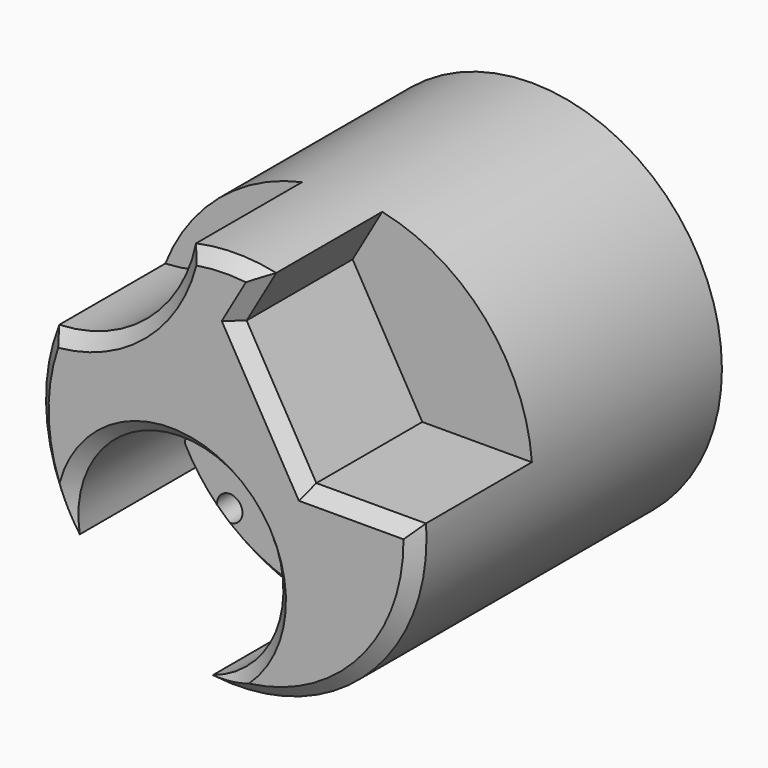
from build123d import *

# Parameters (mm, degrees)
F0_R        = 37.9287365184
F1_DEPTH    = 76.2
F3_R        = 20.4430640503
F4_DEPTH    = 43.688
F5_SIZE     = 2.54
F7_D        = 5.08
F8_T4_ANGLE = 68.0337710329
F8_S5_R     = 20.4430640503
F8_T6_DEPTH = 23


# Not quite as in the source:
# - a fillet or chamfer that OpenCascade refuses, or shapes differently, is made with other operations: its cross-section is extruded or revolved along the edge and cut away or added


with BuildPart() as f1:
    # F0 (on Front) → F1 (new body)
    with BuildSketch(Plane.XZ):
        Circle(F0_R)
    extrude(amount=F1_DEPTH)

    # F3 (on offset) → F4 (cut)
    with BuildSketch(Plane.XZ.offset(47.244)):
        with BuildLine():
            Line((-7.417100016, 52.0775169134), (-39.2948538065, 52.0775169134))
            Line((-39.2948538065, 52.0775169134), (-39.2948538065, 13.8873383403))
            Line((-39.2948538065, 13.8873383403), (-36.437637775, 13.8873383403))
            ThreePointArc((-36.437637775, 13.8873383403), (-15.9170187319, 22.3872570562), (-7.417100016, 42.9078760992))
            Line((-7.417100016, 42.9078760992), (-7.417100016, 52.0775169134))
        make_face()
        Polygon((43.7327071249, 2.8074141011), (57.5817332447, 26.8609896883), (43.6752387942, 50.8813859194), (15.9197182239, 50.8482065633), (2.070692104, 26.794630976), (15.9771865545, 2.7742347449), align=None)
        with Locations((-11.0355066136, -18.2179771364)):
            Circle(F3_R)
    extrude(amount=F4_DEPTH, mode=Mode.SUBTRACT)

    # F5
    f5_edges = [f1.edges().sort_by_distance(p)[0] for p in [
        (25.118202, -76.2, -28.419448),
        (37.902848, -76.2, 1.401132),
        (26.901202, -76.2, 2.787293),
        (9.023939, -76.2, 14.784433),
        (5.030877, -76.2, 31.936005),
        (-0.009512, -76.2, 37.928735),
        (-17.652727, -76.2, 20.787326),
        (-37.679979, -76.2, -4.336848),
        (-0.443827, -76.2, -0.732692),
    ]]
    chamfer(f5_edges, length=F5_SIZE)

    # F7 (through all)
    with Locations(Plane.XZ.offset(47.244)):
        with Locations((-11.6714835167, -7.6255151071), (0, -13.9276552945), (-14.5282614976, -18.8519991934), (-3.3601692412, -24.743270129), (-11.2020578235, -26.739705354), (-22.4352385849, -24.8684193939)):
            Hole(F7_D / 2)

    # F8: chamfer of 2.54 on 1 edges, made by hand


with BuildPart() as f8_tool2:
    # F8_s3 → F8_t4 (revolve)
    with BuildSketch(Plane(origin=(0, 0, 0), x_dir=(0, 1, 0), z_dir=(0.9987962472, 0, 0.0490515704))):
        Polygon((-44.704, -37.9287365184), (-47.244, -35.3887365184), (-47.244, -37.9287365184), align=None)
    revolve(axis=Axis((0, -47.244, 0), (0, 1, 0)), revolution_arc=F8_T4_ANGLE)

    # F8_s5 → F8_t6 (intersect, symmetric)
    with BuildSketch(Plane.XZ.offset(46)):
        with Locations((-11.0355066136, -18.2179771364)):
            Circle(F8_S5_R)
    extrude(amount=F8_T6_DEPTH, both=True, mode=Mode.INTERSECT)


with BuildPart() as f1_1:
    add(f1.part)

    # F8_t1: cut F8_tool2
    add(f8_tool2.part, mode=Mode.SUBTRACT)


solid = f1_1.part
